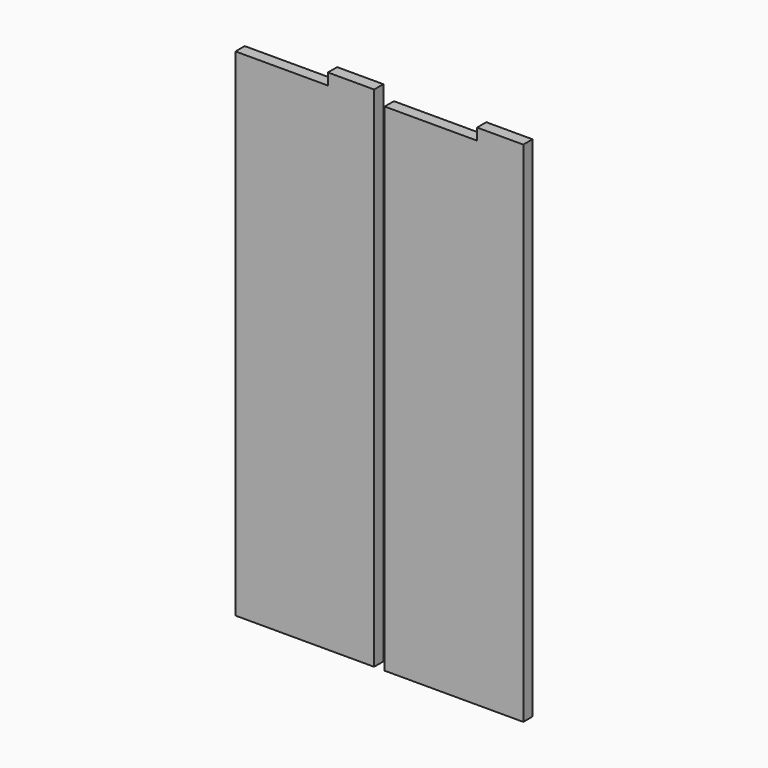
from build123d import *

# Parameters (mm, degrees)
F1_DEPTH = 6.35


# Not quite as in the source:
# - a feature names something its author has since deleted; it is built from what else it names


with BuildPart() as f1:
    # F0 (on Front) → F1 (new body)
    with BuildSketch(Plane.XZ):
        Polygon((345.1327616, -166.950009), (345.1327616, 106.099991), (345.1327616, 112.449991), (319.7327616, 112.449991), (319.7327616, 106.099991), (268.9327616, 106.099991), (268.9327616, -166.950009), align=None)
    extrude(amount=F1_DEPTH)


with BuildPart() as f1b:
    # F0 (on Front) → F1, piece 2 (new body)
    with BuildSketch(Plane.XZ):
        Polygon((263.1353386, -166.950009), (263.1353386, 106.099991), (263.1353386, 112.449991), (237.7353386, 112.449991), (237.7353386, 106.099991), (186.9353386, 106.099991), (186.9353386, -166.950009), align=None)
    extrude(amount=F1_DEPTH)


solid = Compound([f1.part, f1b.part])
